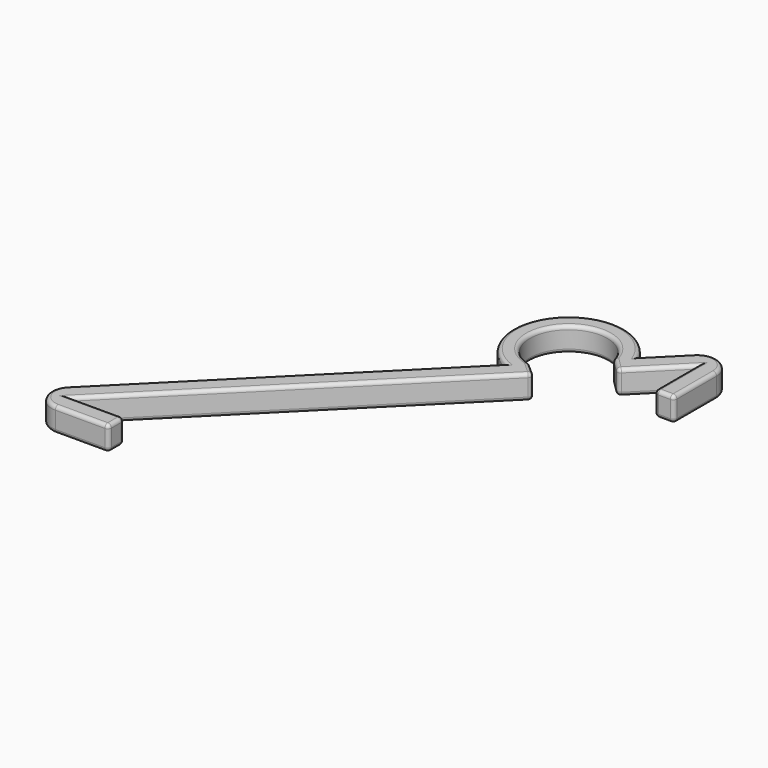
from build123d import *

# Parameters (mm, degrees)
F0_W     = 11
F0_H     = 4
F0_W_2   = 4
F0_H_2   = 11
F1_DEPTH = 5
F2_R     = 0.75


# Not quite as in the source:
# - a feature names something its author has since deleted; it is built from what else it names


with BuildPart() as f1:
    # F0 (on Top) → F1 (new body)
    with BuildSketch(Plane.XY):
        with Locations((-30.5, -38)):
            Rectangle(F0_W, F0_H)
        with Locations((38, 30.5)):
            Rectangle(F0_W_2, F0_H_2)
        with BuildLine():
            Line((-38.8284271247, -33.1715728753), (-36, -36))
            Line((-36, -36), (16.0162036535, 16.0162036535))
            ThreePointArc((16.0162036535, 16.0162036535), (13.656492284, 16.2997541163), (11.4054619105, 17.06231616))
            Line((11.4054619105, 17.06231616), (-38.8284271247, -33.1715728753))
        make_face()
        with BuildLine():
            Line((-36, -40), (-36, -36))
            Line((-36, -36), (-38.8284271247, -33.1715728753))
            ThreePointArc((-38.8284271247, -33.1715728753), (-39.69551813, -37.5307337295), (-36, -40))
        make_face()
        with BuildLine():
            Line((33.1715728753, 38.8284271247), (36, 36))
            Line((36, 36), (40, 36))
            ThreePointArc((40, 36), (37.5307337295, 39.69551813), (33.1715728753, 38.8284271247))
        make_face()
        with BuildLine():
            Line((27.699525099, 27.699525099), (36, 36))
            Line((36, 36), (33.1715728753, 38.8284271247))
            Line((33.1715728753, 38.8284271247), (26.6534125925, 32.310266842))
            ThreePointArc((26.6534125925, 32.310266842), (27.4159746362, 30.0592364686), (27.699525099, 27.699525099))
        make_face()
        with BuildLine():
            ThreePointArc((11.4054619105, 17.06231616), (13.656492284, 16.2997541163), (16.0162036535, 16.0162036535))
            Line((16.0162036535, 16.0162036535), (17.1253699809, 17.1253699809))
            Line((17.1253699809, 17.1253699809), (14.130457766, 19.7873120154))
            Line((14.130457766, 19.7873120154), (11.4054619105, 17.06231616))
        make_face()
        with BuildLine():
            Line((26.7568438618, 26.7568438618), (27.699525099, 27.699525099))
            ThreePointArc((27.699525099, 27.699525099), (27.4159746362, 30.0592364686), (26.6534125925, 32.310266842))
            Line((26.6534125925, 32.310266842), (23.9284167371, 29.5852709866))
            Line((23.9284167371, 29.5852709866), (26.7568438618, 26.7568438618))
        make_face()
        with BuildLine():
            ThreePointArc((26.6534125925, 32.310266842), (8.0692821431, 35.6464466094), (11.4054619105, 17.06231616))
            Line((11.4054619105, 17.06231616), (14.130457766, 19.7873120154))
            ThreePointArc((14.130457766, 19.7873120154), (10.5441558773, 33.1715728753), (23.9284167371, 29.5852709866))
            Line((23.9284167371, 29.5852709866), (26.6534125925, 32.310266842))
        make_face()
    extrude(amount=F1_DEPTH)

    # F2
    f2_edges = [f1.edges().sort_by_distance(p)[0] for p in [
        (-13.711483, -8.054628, 0),
        (29.912493, 35.569347, 0),
        (-13.711483, -8.054628, 5),
        (29.912493, 35.569347, 5),
        (-25, -38, 0),
        (-30.5, -36, 0),
        (-9.437315, -9.437315, 0),
        (15.627914, 18.456341, 0),
        (10.544156, 33.171573, 0),
        (25.34263, 28.171057, 0),
        (31.378422, 31.378422, 0),
        (36, 30.5, 0),
        (38, 25, 0),
        (40, 30.5, 0),
        (37.530734, 39.695518, 0),
        (8.069282, 35.646447, 0),
        (-39.695518, -37.530734, 0),
        (-30.5, -40, 0),
        (36, 30.5, 5),
        (36, 25, 2.5),
        (40, 25, 2.5),
        (38, 25, 5),
        (-9.437315, -9.437315, 5),
        (-30.5, -36, 5),
        (-25, -40, 2.5),
        (-25, -36, 2.5),
        (-25, -38, 5),
        (23.928417, 29.585271, 2.5),
        (26.756844, 26.756844, 2.5),
        (17.12537, 17.12537, 2.5),
        (14.130458, 19.787312, 2.5),
        (8.069282, 35.646447, 5),
        (15.627914, 18.456341, 5),
        (25.34263, 28.171057, 5),
        (10.544156, 33.171573, 5),
        (31.378422, 31.378422, 5),
        (40, 30.5, 5),
        (37.530734, 39.695518, 5),
        (-39.695518, -37.530734, 5),
        (-30.5, -40, 5),
    ]]
    fillet(f2_edges, radius=F2_R)


solid = f1.part
